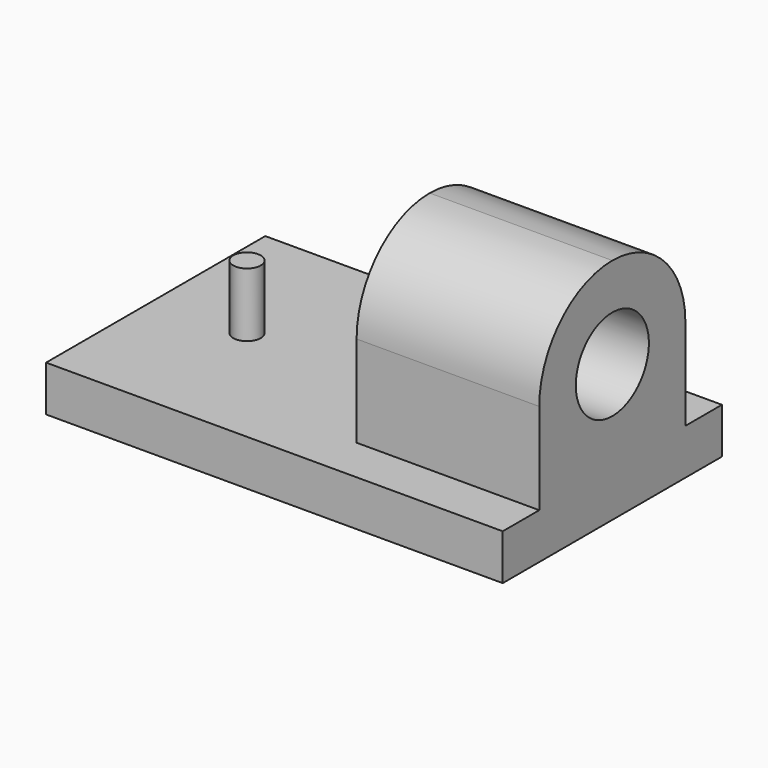
from build123d import *

# Parameters (mm, degrees)
F0_W     = 250
F0_H     = 150
F7_DEPTH = 25
F1_R     = 7.5
F2_DEPTH = 35
F3_W     = 100
F3_H     = 100
F4_DEPTH = 100
F5_R     = 25
F8_DEPTH = 100.001
F6_R     = 49.99999


# Not quite as in the source:
# - a fillet or chamfer is up to 0.001 mm smaller than in the source, because OpenCascade refuses the exact size


with BuildPart() as f7:
    # F0 (on Top) → F7 (new body)
    with BuildSketch(Plane.XY):
        Rectangle(F0_W, F0_H)
    extrude(amount=F7_DEPTH)

    # F1 (on face) → F2 (join)
    with BuildSketch(Plane.XY.offset(25)):
        with Locations((-75, 0)):
            Circle(F1_R)
    extrude(amount=F2_DEPTH)

    # F3 (on face) → F4 (join)
    with BuildSketch(Plane.XY.offset(25)):
        with Locations((75, 0)):
            Rectangle(F3_W, F3_H)
    extrude(amount=F4_DEPTH)

    # F5 (on face) → F8 (cut, through all)
    with BuildSketch(Plane(origin=(25, 0, 0), x_dir=(0, -1, 0), z_dir=(-1, 0, 0))):
        with Locations((0, 75)):
            Circle(F5_R)
    extrude(amount=-F8_DEPTH, mode=Mode.SUBTRACT)

    # F6 (radius 50 in the source; OpenCascade refuses exactly that, so slightly less here)
    f6_edges = [f7.edges().sort_by_distance(p)[0] for p in [
        (75, 50, 125),
        (75, -50, 125),
    ]]
    fillet(f6_edges, radius=F6_R)


solid = f7.part
